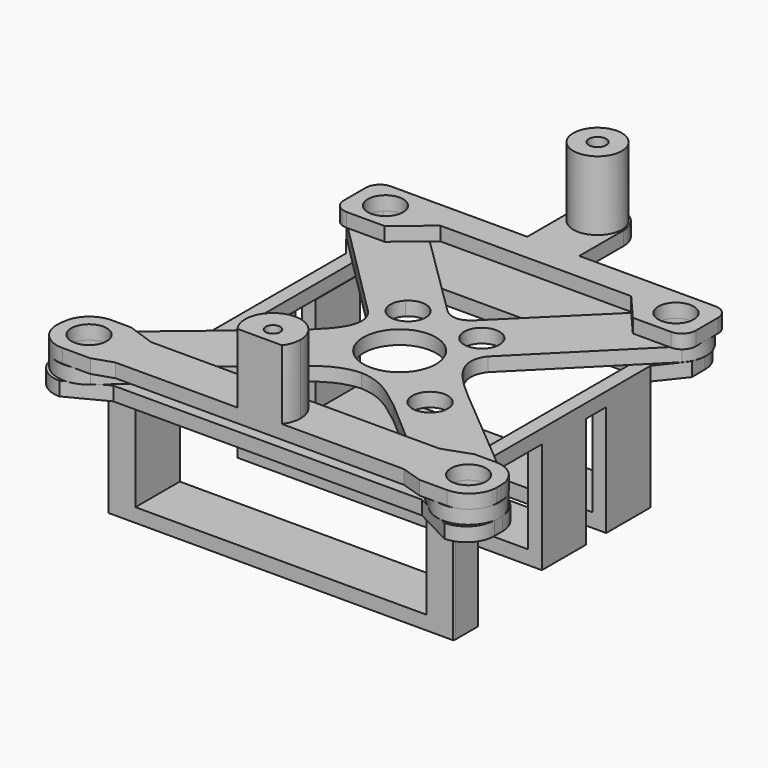
from build123d import *

# Parameters (mm, degrees)
F0_R      = 1.275
F0_R_2    = 2.6199281288
F1_DEPTH  = 1
F2_W      = 19.9647173285
F2_H      = 15.6046988085
F3_DEPTH  = 1
F4_W      = 19.9647173285
F4_H      = 4
F5_DEPTH  = 8
F6_W      = 21
F6_H      = 7.0297351163
F7_DEPTH  = 25
F11_DEPTH = 1
F10_R     = 1.75
F12_D     = 2.55
F12_DEPTH = 9.001
F13_D     = 2.55
F13_2_D   = 2.55
F13_3_D   = 2.55
F9_R      = 0.525
F14_DEPTH = 6
F10_R_2   = 0.625
F4_W_2    = 1
F15_DEPTH = 8


# Not quite as in the source:
# - a feature names something its author has since deleted; it is built from what else it names


with BuildPart() as f1:
    # F0 (on Top) → F1 (new body)
    with BuildSketch(Plane.XY):
        with BuildLine():
            ThreePointArc((-9.573328688, 9.8272704817), (-11.3764239196, 9.8173919204), (-11.3863024809, 11.6204871519))
            Line((-11.3863024809, 11.6204871519), (-12.03834564, 12.2654245841))
            ThreePointArc((-12.03834564, 12.2654245841), (-12.6715211593, 10.7663754037), (-12.0969320414, 9.2439079889))
            Line((-12.0969320414, 9.2439079889), (-8.9526037227, 6.0995796703))
            ThreePointArc((-8.9526037227, 6.0995796703), (-8.091524846, 6.800744053), (-7.2828560364, 7.56175856))
            Line((-7.2828560364, 7.56175856), (-9.573328688, 9.8272704817))
        make_face()
        with BuildLine():
            ThreePointArc((-11.3863024809, 11.6204871519), (-9.9951227915, 11.903157366), (-9.2048155844, 10.7238788168))
            ThreePointArc((-9.2048155844, 10.7238788168), (-9.3005370353, 10.2391860239), (-9.573328688, 9.8272704817))
            Line((-9.573328688, 9.8272704817), (-7.2828560364, 7.56175856))
            ThreePointArc((-7.2828560364, 7.56175856), (-6.5368820612, 8.3715597711), (-5.8502771075, 9.2322738994))
            Line((-5.8502771075, 9.2322738994), (-8.8626991275, 12.2038496447))
            ThreePointArc((-8.8626991275, 12.2038496447), (-10.4373189975, 12.9155843917), (-12.03834564, 12.2654245841))
            Line((-12.03834564, 12.2654245841), (-11.3863024809, 11.6204871519))
        make_face()
        with BuildLine():
            ThreePointArc((-5.8502771075, 9.2322738994), (-6.5368820612, 8.3715597711), (-7.2828560364, 7.56175856))
            ThreePointArc((-7.2828560364, 7.56175856), (-8.091524846, 6.800744053), (-8.9526037227, 6.0995796703))
            Line((-8.9526037227, 6.0995796703), (-4.3187574483, 1.4657333959))
            add(Edge.make_bspline(
                [(-6.5644085681, -3.0918860155), (-4.6455315314, -1.4929088065), (-3.2193431157, 0), (-4.3187574483, 1.4657333959)],
                knots=[0, 0, 0, 0, 5.080831, 5.080831, 5.080831, 5.080831], degree=3))
            Line((-6.5644085681, -3.0918860155), (-14.9908974424, -10.162549722))
            ThreePointArc((-14.9908974424, -10.162549722), (-15.4591160696, -13.3890767422), (-12.2139242893, -13.7028212304))
            Line((-12.2139242893, -13.7028212304), (-3.8926461712, -6.50863396))
            add(Edge.make_bspline(
                [(-3.8926461712, -6.50863396), (-2.5926211856, -5.5163033886), (-1.6234933864, -4.629815463), (0, -4.5469403267)],
                knots=[0, 0, 0, 0, 4.3590063231, 4.3590063231, 4.3590063231, 4.3590063231], degree=3))
            add(Edge.make_bspline(
                [(3.8926461712, -6.50863396), (2.5926211856, -5.5163033886), (1.6234933864, -4.629815463), (0, -4.5469403267)],
                knots=[0, 0, 0, 0, 4.3590063231, 4.3590063231, 4.3590063231, 4.3590063231], degree=3))
            Line((3.8926461712, -6.50863396), (12.2139242893, -13.7028212304))
            ThreePointArc((12.2139242893, -13.7028212304), (15.4591160696, -13.3890767422), (14.9908974424, -10.162549722))
            Line((14.9908974424, -10.162549722), (6.5644085681, -3.0918860155))
            add(Edge.make_bspline(
                [(6.5644085681, -3.0918860155), (4.6455315314, -1.4929088065), (3.2193431157, 0), (4.3187574483, 1.4657333959)],
                knots=[0, 0, 0, 0, 5.080831, 5.080831, 5.080831, 5.080831], degree=3))
            Line((4.3187574483, 1.4657333959), (12.0969320414, 9.2439079889))
            ThreePointArc((12.0969320414, 9.2439079889), (11.9597864123, 12.3409952738), (8.8626991275, 12.2038496447))
            Line((8.8626991275, 12.2038496447), (1.0316137923, 4.4789481908))
            add(Edge.make_bspline(
                [(-1.0316137923, 4.4789481908), (-0.3709533485, 3.8162749261), (0.3629251732, 3.8162749261), (1.0316137923, 4.4789481908)],
                knots=[0, 0, 0, 0, 2.0632275846, 2.0632275846, 2.0632275846, 2.0632275846], degree=3))
            Line((-1.0316137923, 4.4789481908), (-5.8502771075, 9.2322738994))
        make_face()
        with BuildLine():
            ThreePointArc((-12.4119621518, -11.9990071271), (-14.8850880719, -12.4350338232), (-12.7101884728, -11.1795327956))
            ThreePointArc((-12.7101884728, -11.1795327956), (-12.4888362317, -11.5629804311), (-12.4119621518, -11.9990071271))
        make_face(mode=Mode.SUBTRACT)
        with BuildLine():
            ThreePointArc((-6.2366687965, -5.7485068336), (-5.6959218136, -3.7309065819), (-3.9848951175, -4.929032502))
            ThreePointArc((-3.9848951175, -4.929032502), (-4.8238684215, -6.1271584221), (-6.2366687965, -5.7485068336))
        make_face(mode=Mode.SUBTRACT)
        with Locations((13.6869621518, -11.9990071271)):
            Circle(F0_R, mode=Mode.SUBTRACT)
        with Locations((5.2598951175, -4.929032502)):
            Circle(F0_R, mode=Mode.SUBTRACT)
        with Locations((0, -1.0985087138)):
            Circle(F0_R_2, mode=Mode.SUBTRACT)
        with BuildLine():
            ThreePointArc((-1.3841443211, 2.9884343571), (-3.143837114, 1.8091558079), (-3.5656312175, 3.8850426922))
            ThreePointArc((-3.5656312175, 3.8850426922), (-2.1744515281, 4.1677129062), (-1.3841443211, 2.9884343571))
        make_face(mode=Mode.SUBTRACT)
        with Locations((2.6591443211, 2.9884343571)):
            Circle(F0_R, mode=Mode.SUBTRACT)
        with Locations((10.4798155844, 10.7238788168)):
            Circle(F0_R, mode=Mode.SUBTRACT)
    extrude(amount=F1_DEPTH)


with BuildPart() as f3:
    # F2 (on Top) → F3 (new body)
    with BuildSketch(Plane.XY):
        with BuildLine():
            Line((-11.1375301927, -13), (11.1375301927, -13))
            Line((11.1375301927, -13), (13.8875301927, -14.4273526967))
            ThreePointArc((13.8875301927, -14.4273526967), (15.3017437551, -13.841566259), (15.8875301927, -12.4273526967))
            Line((15.8875301927, -12.4273526967), (15.8875301927, -11.6773526967))
            ThreePointArc((15.8875301927, -11.6773526967), (15.3017437551, -10.2631391343), (13.8875301927, -9.6773526967))
            Line((13.8875301927, -9.6773526967), (12.5374241024, -9.6773526967))
            Line((12.5374241024, -9.6773526967), (12.4625758976, -9.6773526967))
            Line((12.4625758976, -9.6773526967), (12.4625758976, -9.5891059329))
            Line((12.4625758976, -9.5891059329), (10.9823586643, -7.8439153731))
            Line((10.9823586643, -7.8439153731), (10.9823586643, 7.8023494042))
            Line((10.9823586643, 7.8023494042), (12.4625758976, 9.6674818319))
            Line((12.4625758976, 9.6674818319), (12.4625758976, 10.8503765091))
            ThreePointArc((12.4625758976, 10.8503765091), (11.8767894599, 12.2645900715), (10.4625758976, 12.8503765091))
            Line((10.4625758976, 12.8503765091), (-10.5374241024, 12.8503765091))
            ThreePointArc((-10.5374241024, 12.8503765091), (-11.9516376648, 12.2645900715), (-12.5374241024, 10.8503765091))
            Line((-12.5374241024, 10.8503765091), (-12.5374241024, 9.7617935389))
            Line((-12.5374241024, 9.7617935389), (-10.9823586643, 7.8023494042))
            Line((-10.9823586643, 7.8023494042), (-10.9823586643, -7.8439153731))
            Line((-10.9823586643, -7.8439153731), (-12.5374241024, -9.6773526967))
            Line((-12.5374241024, -9.6773526967), (-13.8875301927, -9.6773526967))
            ThreePointArc((-13.8875301927, -9.6773526967), (-15.3017437551, -10.2631391343), (-15.8875301927, -11.6773526967))
            Line((-15.8875301927, -11.6773526967), (-15.8875301927, -12.4273526967))
            ThreePointArc((-15.8875301927, -12.4273526967), (-15.3017437551, -13.841566259), (-13.8875301927, -14.4273526967))
            Line((-13.8875301927, -14.4273526967), (-11.1375301927, -13))
        make_face()
        Rectangle(F2_W, F2_H, mode=Mode.SUBTRACT)
    extrude(amount=-F3_DEPTH)

    # F4 (on face) → F5 (join)
    with BuildSketch(Plane(origin=(0, 0, -1), x_dir=(1, 0, 0), z_dir=(0, 0, -1))):
        Polygon((-9.9823586643, 7.8023494042), (9.9823586643, 7.8023494042), (10.9823586643, 7.8023494042), (10.9823586643, 7.8439153731), (12.4625758976, 9.5891059329), (12.4625758976, 9.6773526967), (12.4625758976, 11.8023494042), (-12.4625758976, 11.8023494042), (-12.4625758976, 9.5891059329), (-10.9823586643, 7.8439153731), (-10.9823586643, 7.8023494042), align=None)
        Rectangle(F4_W, F4_H)
        with Locations((0, -5.8023494042)):
            Rectangle(F4_W, F4_H)
    extrude(amount=F5_DEPTH)

    # F6 (on face) → F7 (cut)
    with BuildSketch(Plane.XZ.offset(11.8023494042)):
        with Locations((0, -4.4851324419)):
            Rectangle(F6_W, F6_H)
    extrude(amount=-F7_DEPTH, mode=Mode.SUBTRACT)

    # F12 (through all, one way)
    with BuildSketch(Plane.XY):
        with Locations((-13.6869621518, -11.9990071271), (13.6869621518, -11.9990071271), (10.4798155844, 10.7238788168), (-10.4798155844, 10.7238788168)):
            Circle(F12_D / 2)
    extrude(amount=-F12_DEPTH, mode=Mode.SUBTRACT)

    # F4 (on face) → F15 (join)
    with BuildSketch(Plane(origin=(0, 0, -1), x_dir=(1, 0, 0), z_dir=(0, 0, -1))):
        with Locations((10.4823586643, -5.8023494042)):
            Rectangle(F4_W_2, F4_H)
        with Locations((10.4823586643, 0)):
            Rectangle(F4_W_2, F4_H)
        with Locations((-10.4823586643, 0)):
            Rectangle(F4_W_2, F4_H)
        with Locations((-10.4823586643, -5.8023494042)):
            Rectangle(F4_W_2, F4_H)
    extrude(amount=F15_DEPTH)


with BuildPart() as f11:
    # F9 (on offset) → F11 (new body)
    with BuildSketch(Plane.XY.offset(1)):
        with BuildLine():
            Line((-12.3886769961, -9.8252212629), (-13.8104255105, -9.8252212629))
            ThreePointArc((-13.8104255105, -9.8252212629), (-15.1393509349, -10.3305784239), (-15.7966943797, -11.5912640467))
            Line((-15.7966943797, -11.5912640467), (-15.8405235187, -11.9633682104))
            ThreePointArc((-15.8405235187, -11.9633682104), (-15.3488974884, -13.526250851), (-13.8542546494, -14.1973254265))
            Line((-13.8542546494, -14.1973254265), (-11.8422154016, -14.1973254265))
            Line((-11.8422154016, -14.1973254265), (-10.4036418671, -13.7202938231))
            Line((-10.4036418671, -13.7202938231), (-1.6026274117, -13.7202938231))
            ThreePointArc((-1.6026274117, -13.7202938231), (-1.7878726943, -11.6274171734), (0, -10.523805052))
            Line((0, -10.523805052), (-10.4036418671, -10.523805052))
            Line((-10.4036418671, -10.523805052), (-12.3886769961, -9.8252212629))
        make_face()
    extrude(amount=F11_DEPTH)

    # F13 (through all)
    with Locations(Plane(origin=(0, 0, 0), x_dir=(1, 0, 0), z_dir=(0, 0, -1))):
        with Locations((-13.6869621518, 11.9990071271), (13.6869621518, 11.9990071271), (-10.4798155844, -10.7238788168), (10.4798155844, -10.7238788168)):
            Hole(F13_D / 2)



with BuildPart() as f11b:
    # F9 (on offset) → F11, piece 2 (new body)
    with BuildSketch(Plane.XY.offset(1)):
        with BuildLine():
            Line((10.4036418671, -10.523805052), (0, -10.523805052))
            ThreePointArc((0, -10.523805052), (1.4142135624, -11.1095914897), (2, -12.523805052))
            ThreePointArc((2, -12.523805052), (1.8980588536, -13.1541800106), (1.6026274117, -13.7202938231))
            Line((1.6026274117, -13.7202938231), (10.4036418671, -13.7202938231))
            Line((10.4036418671, -13.7202938231), (11.9101134234, -14.1973254265))
            Line((11.9101134234, -14.1973254265), (13.8957873518, -14.1973254265))
            ThreePointArc((13.8957873518, -14.1973254265), (15.3100009142, -13.6115389889), (15.8957873518, -12.1973254265))
            Line((15.8957873518, -12.1973254265), (15.8957873518, -11.8252212629))
            ThreePointArc((15.8957873518, -11.8252212629), (15.3100009142, -10.4110077005), (13.8957873518, -9.8252212629))
            Line((13.8957873518, -9.8252212629), (12.3886769961, -9.8252212629))
            Line((12.3886769961, -9.8252212629), (10.4036418671, -10.523805052))
        make_face()
    extrude(amount=F11_DEPTH)

    # F13#2 (through all)
    with Locations(Plane(origin=(0, 0, 0), x_dir=(1, 0, 0), z_dir=(0, 0, -1))):
        with Locations((-13.6869621518, 11.9990071271), (13.6869621518, 11.9990071271), (-10.4798155844, -10.7238788168), (10.4798155844, -10.7238788168)):
            Hole(F13_2_D / 2)


with BuildPart() as f11c:
    # F10 (on offset) → F11, piece 3 (new body)
    with BuildSketch(Plane.XY.offset(1)):
        with BuildLine():
            Line((-1.875, 12.7523494042), (-11.7122084051, 12.7523494042))
            ThreePointArc((-11.7122084051, 12.7523494042), (-12.4193151863, 12.4594561854), (-12.7122084051, 11.7523494042))
            Line((-12.7122084051, 11.7523494042), (-12.7122084051, 9.7523494042))
            ThreePointArc((-12.7122084051, 9.7523494042), (-12.4193151863, 9.0452426231), (-11.7122084051, 8.7523494042))
            Line((-11.7122084051, 8.7523494042), (-8.9622084051, 8.7523494042))
            Line((-8.9622084051, 8.7523494042), (-6.5461620688, 10.7523494042))
            Line((-6.5461620688, 10.7523494042), (7.2237383574, 10.7523494042))
            Line((7.2237383574, 10.7523494042), (8.9398968592, 8.7523494042))
            Line((8.9398968592, 8.7523494042), (11.6898968592, 8.7523494042))
            ThreePointArc((11.6898968592, 8.7523494042), (12.3970036404, 9.0452426231), (12.6898968592, 9.7523494042))
            Line((12.6898968592, 9.7523494042), (12.6898968592, 11.7523494042))
            ThreePointArc((12.6898968592, 11.7523494042), (12.3970036404, 12.4594561854), (11.6898968592, 12.7523494042))
            Line((11.6898968592, 12.7523494042), (1.875, 12.7523494042))
            Line((1.875, 12.7523494042), (1.875, 16.7523494042))
            ThreePointArc((1.875, 16.7523494042), (0, 18.6273494042), (-1.875, 16.7523494042))
            Line((-1.875, 16.7523494042), (-1.875, 12.7523494042))
        make_face()
        with Locations((0, 16.7523494042)):
            Circle(F10_R, mode=Mode.SUBTRACT)
    extrude(amount=F11_DEPTH)

    # F13#3 (through all)
    with Locations(Plane(origin=(0, 0, 0), x_dir=(1, 0, 0), z_dir=(0, 0, -1))):
        with Locations((-13.6869621518, 11.9990071271), (13.6869621518, 11.9990071271), (-10.4798155844, -10.7238788168), (10.4798155844, -10.7238788168)):
            Hole(F13_3_D / 2)

    # F10 (on offset) → F14, piece 2 (join)
    with BuildSketch(Plane.XY.offset(1)):
        with Locations((0, 16.7523494042)):
            Circle(F10_R)
        with Locations((0, 16.7523494042)):
            Circle(F10_R_2, mode=Mode.SUBTRACT)
    extrude(amount=F14_DEPTH)


with BuildPart() as f11_1:
    add(f11.part)

    add(f11b.part)  # F14 merges F11b
    # F9 (on offset) → F14 (join)
    with BuildSketch(Plane.XY.offset(1)):
        with BuildLine():
            ThreePointArc((2, -12.523805052), (1.4142135624, -11.1095914897), (0, -10.523805052))
            ThreePointArc((0, -10.523805052), (-1.7878726943, -11.6274171734), (-1.6026274117, -13.7202938231))
            Line((-1.6026274117, -13.7202938231), (0, -13.7202938231))
            Line((0, -13.7202938231), (1.6026274117, -13.7202938231))
            ThreePointArc((1.6026274117, -13.7202938231), (1.8980588536, -13.1541800106), (2, -12.523805052))
        make_face()
        with Locations((0, -12.523805052)):
            Circle(F9_R, mode=Mode.SUBTRACT)
    extrude(amount=F14_DEPTH)


solid = Compound([f1.part, f3.part, f11c.part, f11_1.part])
